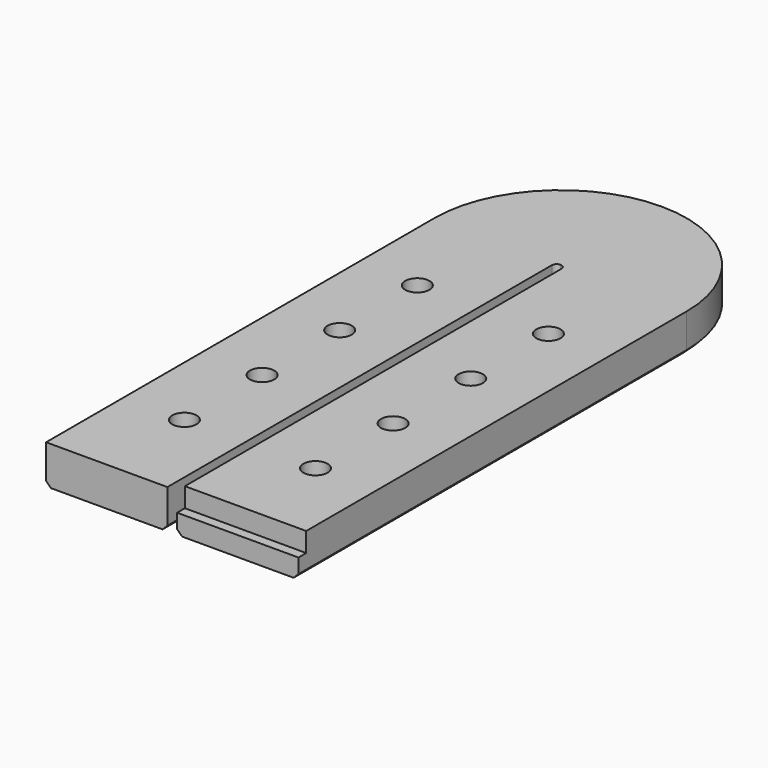
from build123d import *

# Parameters (mm, degrees)
F0_R     = 125
F1_DEPTH = 400
F0_W     = 1250
F0_H     = 100
F2_DEPTH = 200
F3_SIZE  = 50
F4_R     = 49.99999


# Not quite as in the source:
# - a fillet or chamfer is up to 0.001 mm smaller than in the source, because OpenCascade refuses the exact size


with BuildPart() as f1:
    # F0 (on Top) → F1 (new body)
    with BuildSketch(Plane.XY):
        with BuildLine():
            Line((-50, 0), (0, 0))
            Line((0, 0), (50, 0))
            Line((50, 0), (50, -4900))
            Line((50, -4900), (1300, -4900))
            Line((1300, -4900), (1300, 0))
            ThreePointArc((1300, 0), (0, 1300), (-1300, 0))
            Line((-1300, 0), (-1300, -5000))
            Line((-1300, -5000), (-50, -5000))
            Line((-50, -5000), (-50, 0))
        make_face()
        with Locations((-675, -4000)):
            Circle(F0_R, mode=Mode.SUBTRACT)
        with Locations((-675, -3000)):
            Circle(F0_R, mode=Mode.SUBTRACT)
        with Locations((-675, -2000)):
            Circle(F0_R, mode=Mode.SUBTRACT)
        with Locations((675, -4000)):
            Circle(F0_R, mode=Mode.SUBTRACT)
        with Locations((675, -3000)):
            Circle(F0_R, mode=Mode.SUBTRACT)
        with Locations((675, -2000)):
            Circle(F0_R, mode=Mode.SUBTRACT)
        with Locations((-675, -1000)):
            Circle(F0_R, mode=Mode.SUBTRACT)
        with Locations((675, -1000)):
            Circle(F0_R, mode=Mode.SUBTRACT)
    extrude(amount=F1_DEPTH)

    # F0 (on Top) → F2 (join)
    with BuildSketch(Plane.XY):
        with Locations((675, -4950)):
            Rectangle(F0_W, F0_H)
    extrude(amount=F2_DEPTH)

    # F3
    f3_edges = [f1.edges().sort_by_distance(p)[0] for p in [
        (-1300, -2500, 0),
        (0, 1300, 0),
        (1300, -2500, 0),
        (-50, -2500, 0),
        (50, -2500, 0),
        (0, 0, 0),
    ]]
    chamfer(f3_edges, length=F3_SIZE)

    # F4 (radius 50 in the source; OpenCascade refuses exactly that, so slightly less here)
    f4_edges = [f1.edges().sort_by_distance(p)[0] for p in [
        (50, 0, 225),
        (-50, 0, 225),
    ]]
    fillet(f4_edges, radius=F4_R)


solid = f1.part
